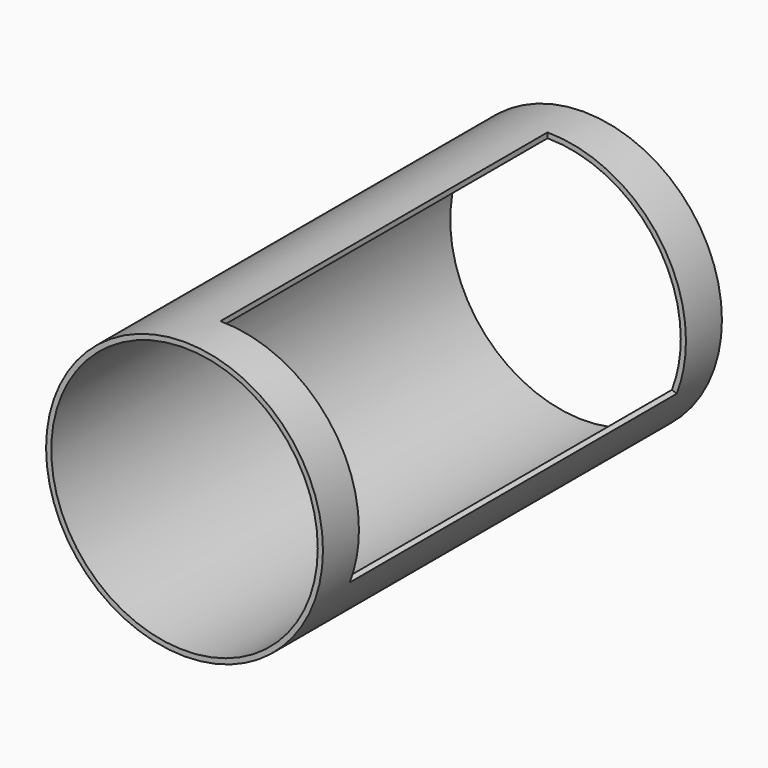
from build123d import *

# Parameters (mm, degrees)
F0_R     = 254
F0_R_2   = 244.5
F1_DEPTH = 457.5
F3_DEPTH = 375


with BuildPart() as f1:
    # F0 (on Front) → F1 (new body, symmetric)
    with BuildSketch(Plane.XZ):
        Circle(F0_R)
        Circle(F0_R_2, mode=Mode.SUBTRACT)
    extrude(amount=F1_DEPTH, both=True)

    # F2 (on Front) → F3 (cut, symmetric)
    with BuildSketch(Plane.XZ):
        with BuildLine():
            ThreePointArc((237.1294283303, -91.0254591845), (209.32805191, 143.8671841789), (0, 254))
            Line((0, 254), (0, 244.5))
            ThreePointArc((0, 244.5), (201.4988531181, 138.4863249281), (228.2604142786, -87.6209636638))
            Line((228.2604142786, -87.6209636638), (237.1294283303, -91.0254591845))
        make_face()
        with BuildLine():
            ThreePointArc((228.2604142786, -87.6209636638), (201.4988531181, 138.4863249281), (0, 244.5))
            Line((0, 244.5), (0, 0))
            Line((0, 0), (228.2604142786, -87.6209636638))
        make_face()
    extrude(amount=F3_DEPTH, both=True, mode=Mode.SUBTRACT)


solid = f1.part
